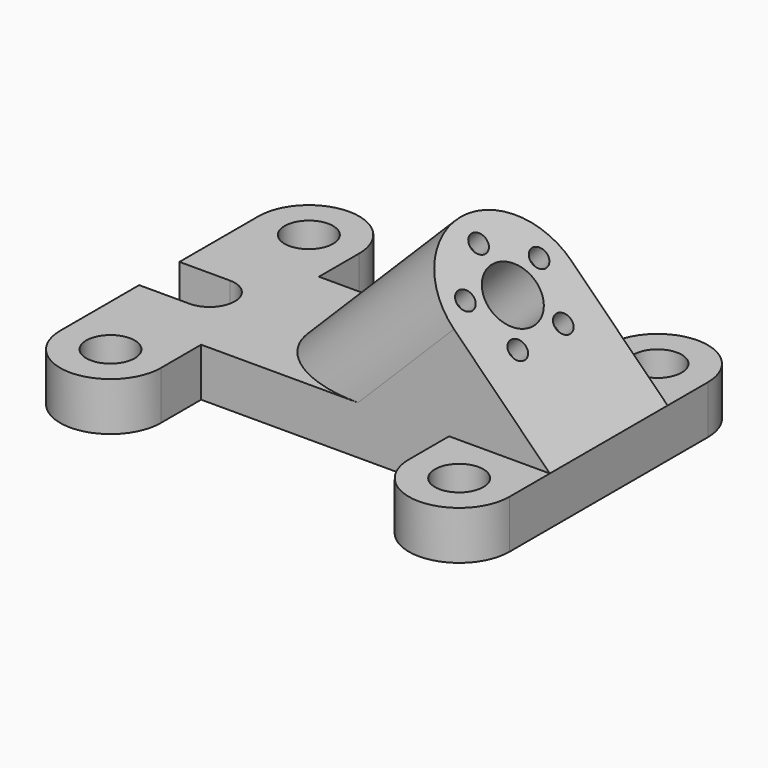
from build123d import *

# Parameters (mm, degrees)
F0_R     = 6.25
F1_DEPTH = 12.5
F3_DEPTH = 38
F4_R     = 18.99999
F5_R     = 2.5
F6_DEPTH = 5
F7_R     = 7.5
F8_DEPTH = 100


# Not quite as in the source:
# - a fillet or chamfer is up to 0.001 mm smaller than in the source, because OpenCascade refuses the exact size


with BuildPart() as f1:
    # F0 (on Top) → F1 (new body)
    with BuildSketch(Plane.XY):
        with BuildLine():
            Line((-13, 25.5), (-13, 0))
            ThreePointArc((-13, 0), (0, -13), (13, 0))
            Line((13, 0), (13, 13))
            Line((13, 13), (77, 13))
            Line((77, 13), (77, 0))
            ThreePointArc((77, 0), (90, -13), (103, 0))
            Line((103, 0), (103, 64))
            ThreePointArc((103, 64), (90, 77), (77, 64))
            Line((77, 64), (77, 51))
            Line((77, 51), (13, 51))
            Line((13, 51), (13, 64))
            ThreePointArc((13, 64), (0, 77), (-13, 64))
            Line((-13, 64), (-13, 38.5))
            Line((-13, 38.5), (0, 38.5))
            ThreePointArc((0, 38.5), (6.5, 32), (0, 25.5))
            Line((0, 25.5), (-13, 25.5))
        make_face()
        Circle(F0_R, mode=Mode.SUBTRACT)
        with Locations((90, 0)):
            Circle(F0_R, mode=Mode.SUBTRACT)
        with Locations((0, 64)):
            Circle(F0_R, mode=Mode.SUBTRACT)
        with Locations((90, 64)):
            Circle(F0_R, mode=Mode.SUBTRACT)
    extrude(amount=F1_DEPTH)

    # F2 (on face) → F3 (join)
    with BuildSketch(Plane.XZ.offset(-13)):
        Polygon((26.6324676319, 12.5), (77, 12.5), (103, 12.5), (64.8162338159, 50.6837661841), align=None)
    extrude(amount=-F3_DEPTH)

    # F4 (radius 19 in the source; OpenCascade refuses exactly that, so slightly less here)
    f4_edges = [f1.edges().sort_by_distance(p)[0] for p in [
        (45.724351, 13, 31.591883),
        (45.724351, 51, 31.591883),
    ]]
    fillet(f4_edges, radius=F4_R)

    # F5 (on face) → F6 (cut)
    with BuildSketch(Plane(origin=(57.75, 0, 57.75), x_dir=(0.7071067812, 0, -0.7071067812), z_dir=(0.7071067812, 0, 0.7071067812))):
        with Locations((25.1304512677, 20.1117935463)):
            Circle(F5_R)
        with Locations((39.1058761271, 24.6526843463)):
            Circle(F5_R)
        with Locations((39.1058761271, 39.3473156537)):
            Circle(F5_R)
        with Locations((25.1304512677, 43.8882064537)):
            Circle(F5_R)
        with Locations((16.4931636974, 32)):
            Circle(F5_R)
    extrude(amount=-F6_DEPTH, mode=Mode.SUBTRACT)

    # F7 (on face) → F8 (cut)
    with BuildSketch(Plane(origin=(57.75, 0, 57.75), x_dir=(0.7071067812, 0, -0.7071067812), z_dir=(0.7071067812, 0, 0.7071067812))):
        with Locations((28.9931636974, 32)):
            Circle(F7_R)
    extrude(amount=-F8_DEPTH, mode=Mode.SUBTRACT)


solid = f1.part
